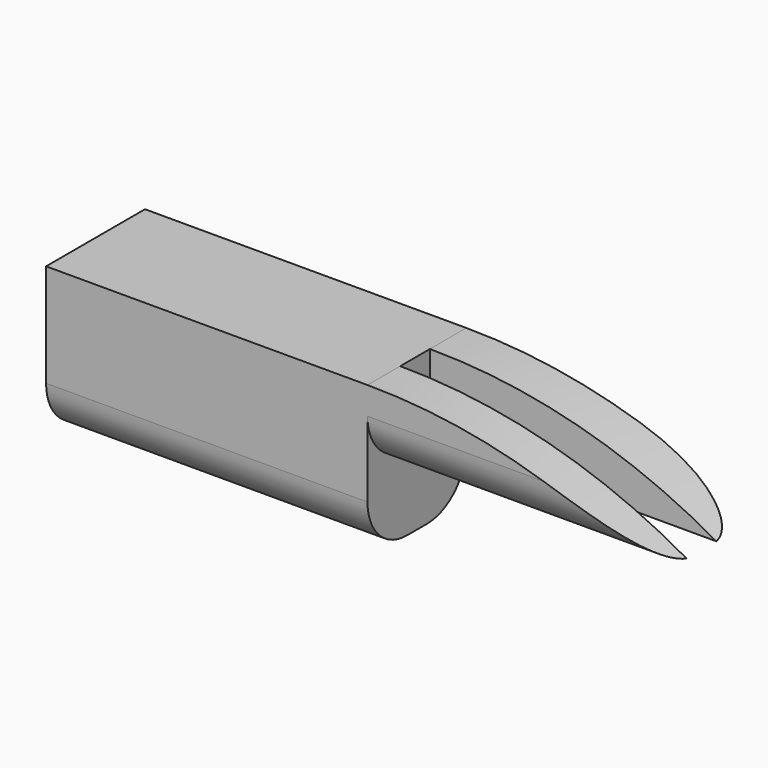
from build123d import *

# Parameters (mm, degrees)
F1_DEPTH    = 12.7
F2_W        = 29.4221741813
F2_H        = 3.8190931082
F3_DEPTH    = 25.4
F4_T1_DEPTH = 58.42
F4_T3_DEPTH = 41.9312775373
F4_T5_DEPTH = 42.0824239574


# Not quite as in the source:
# - a fillet or chamfer that OpenCascade refuses, or shapes differently, is made with other operations: its cross-section is extruded or revolved along the edge and cut away or added


with BuildPart() as f1:
    # F0 (on Front) → F1 (new body)
    with BuildSketch(Plane.XZ):
        Polygon((6.3818255705, 18.0452149361), (-26.6381744295, 18.0452149361), (-26.6381744295, 2.3869331926), (6.3818255705, 2.3869331926), (6.3818255705, 10.2160740644), align=None)
        with BuildLine():
            ThreePointArc((35.8039997518, 10.2160740644), (21.6048326678, 16.0544570681), (6.3818255705, 18.0452149361))
            Line((6.3818255705, 18.0452149361), (6.3818255705, 10.2160740644))
            Line((6.3818255705, 10.2160740644), (35.8039997518, 10.2160740644))
        make_face()
    extrude(amount=F1_DEPTH)

    # F2 (on face) → F3 (cut)
    with BuildSketch(Plane(origin=(0, 0, 10.2160740644), x_dir=(1, 0, 0), z_dir=(0, 0, -1))):
        with Locations((21.0929126611, 6.5879346803)):
            Rectangle(F2_W, F2_H)
    extrude(amount=-F3_DEPTH, mode=Mode.SUBTRACT)

    # F4: fillet of radius 5.08 on 4 edges, made by hand

    # F4_s2 → F4_t1 (cut)
    with BuildSketch(Plane.YZ.offset(-39.3381744295)):
        with BuildLine():
            ThreePointArc((-12.7, 7.4669331926), (-11.2121024484, 3.8748307442), (-7.62, 2.3869331926))
            Line((-7.62, 2.3869331926), (-12.7, 2.3869331926))
            Line((-12.7, 2.3869331926), (-12.7, 7.4669331926))
        make_face()
        with BuildLine():
            ThreePointArc((0, 7.4669331926), (-1.4878975516, 3.8748307442), (-5.08, 2.3869331926))
            Line((-5.08, 2.3869331926), (0, 2.3869331926))
            Line((0, 2.3869331926), (0, 7.4669331926))
        make_face()
    extrude(amount=F4_T1_DEPTH, mode=Mode.SUBTRACT)

    # F4_s4 → F4_t3 (cut)
    with BuildSketch(Plane.YZ.offset(6.3818255705)):
        with BuildLine():
            ThreePointArc((-12.7, 15.2197154068), (-11.5099874467, 11.9525457349), (-8.4974812344, 10.2160740644))
            Line((-8.4974812344, 10.2160740644), (-12.7, 10.2160740644))
            Line((-12.7, 10.2160740644), (-12.7, 15.2197154068))
        make_face()
    extrude(amount=F4_T3_DEPTH, mode=Mode.SUBTRACT)

    # F4_s6 → F4_t5 (cut)
    with BuildSketch(Plane.YZ.offset(6.3818255705)):
        with BuildLine():
            ThreePointArc((0, 15.2801739748), (-1.3486069412, 11.8329858685), (-4.6783881262, 10.2160740644))
            Line((-4.6783881262, 10.2160740644), (0, 10.2160740644))
            Line((0, 10.2160740644), (0, 15.2801739748))
        make_face()
    extrude(amount=F4_T5_DEPTH, mode=Mode.SUBTRACT)


solid = f1.part
